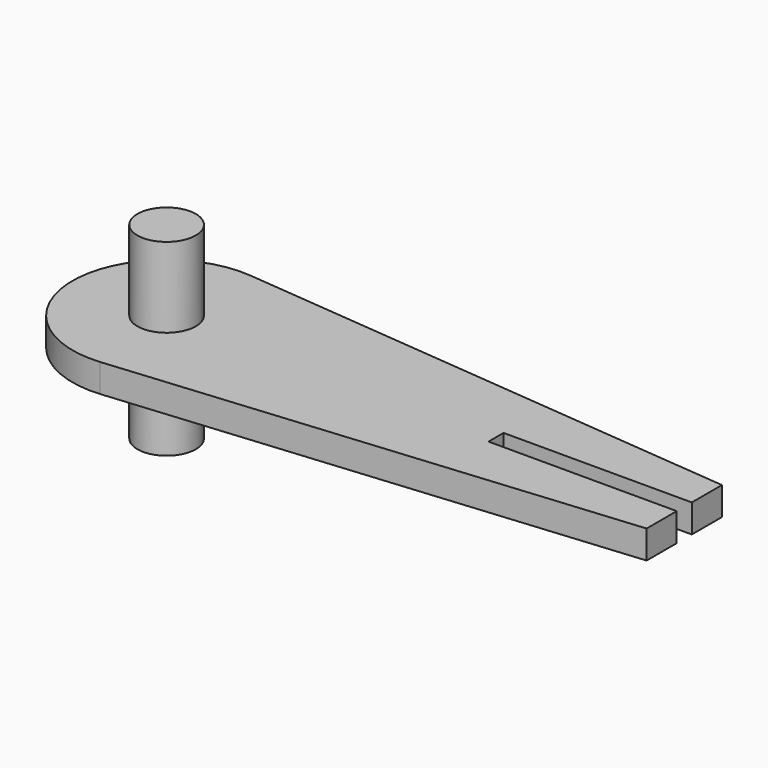
from build123d import *

# Parameters (mm, degrees)
F0_R     = 3.1
F1_DEPTH = 10
F2_DEPTH = 1.5
F3_W     = 20
F3_H     = 2
F4_DEPTH = 11.501


# Not quite as in the source:
# - a feature names something its author has since deleted; it is built from what else it names


with BuildPart() as f1:
    # F0 (on Top) → F1 (new body, symmetric)
    with BuildSketch(Plane.XY):
        Circle(F0_R)
    extrude(amount=F1_DEPTH, both=True)

    # F0 (on Top) → F2 (join, symmetric)
    with BuildSketch(Plane.XY):
        with BuildLine():
            ThreePointArc((0.9128866521, -9.9582447229), (7.3867742121, -6.7405909785), (10, 0))
            ThreePointArc((10, 0), (7.3867742121, 6.7405909785), (0.9128866521, 9.9582447229))
            ThreePointArc((0.9128866521, 9.9582447229), (-10, 0), (0.9128866521, -9.9582447229))
        make_face()
        Circle(F0_R, mode=Mode.SUBTRACT)
        with BuildLine():
            ThreePointArc((0.9128866521, 9.9582447229), (7.3867742121, 6.7405909785), (10, 0))
            ThreePointArc((10, 0), (7.3867742121, -6.7405909785), (0.9128866521, -9.9582447229))
            Line((0.9128866521, -9.9582447229), (55, -5))
            Line((55, -5), (55, 5))
            Line((55, 5), (0.9128866521, 9.9582447229))
        make_face()
    extrude(amount=F2_DEPTH, both=True)

    # F3 (on face) → F4 (cut, through all)
    with BuildSketch(Plane.XY.offset(1.5)):
        with Locations((45, 0)):
            Rectangle(F3_W, F3_H)
    extrude(amount=-F4_DEPTH, mode=Mode.SUBTRACT)


solid = f1.part
